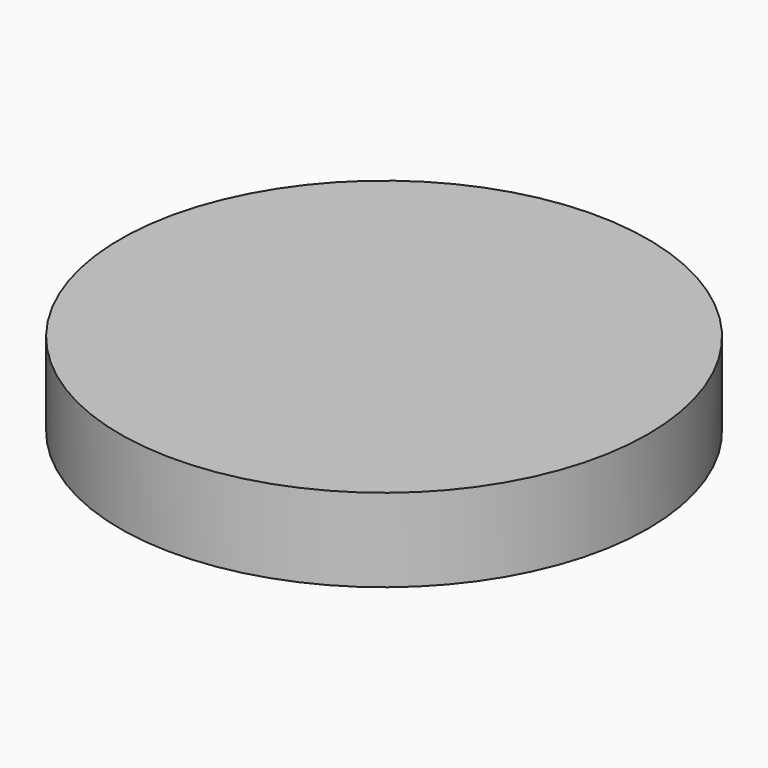
from build123d import *

# Parameters (mm, degrees)
F0_R     = 40.3009330014
F1_DEPTH = 12.7


# Not quite as in the source:
# - the program builds the solid bodies; features that only make, move or delete a surface that nothing else refers to are left out


with BuildPart() as f1:
    # F0 (on Top) → F1 (new body)
    with BuildSketch(Plane.XY):
        with Locations((12.3301092535, 16.3369756192)):
            Circle(F0_R)
    extrude(amount=F1_DEPTH)


solid = f1.part
